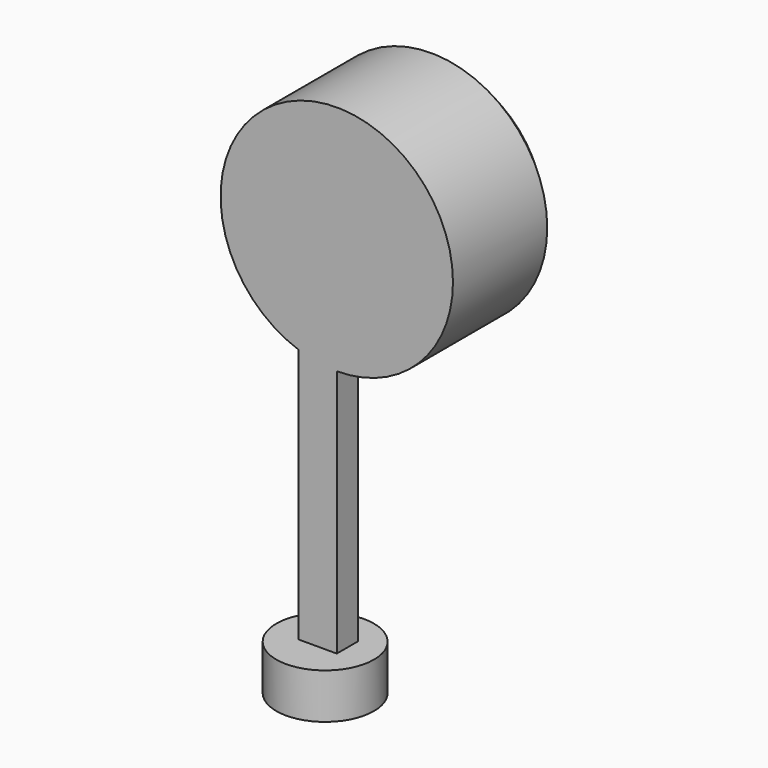
from build123d import *

# Parameters (mm, degrees)
F0_R     = 27.3478618837
F1_DEPTH = 25.4
F2_W     = 21.4937683195
F2_H     = 14.953751117
F3_DEPTH = 228.6
F4_R     = 65.1026145731
F5_DEPTH = 76.2
F6_R     = 40.595906751
F7_DEPTH = 25.4
F8_R     = 12.7


# Not quite as in the source:
# - a fillet or chamfer that OpenCascade refuses, or shapes differently, is made with other operations: its cross-section is extruded or revolved along the edge and cut away or added


with BuildPart() as f1:
    # F0 (on Top) → F1 (new body)
    with BuildSketch(Plane.XY):
        with Locations((-20.4128082842, 28.926692903)):
            Circle(F0_R)
    extrude(amount=F1_DEPTH)

    # F2 (on face) → F3 (join)
    with BuildSketch(Plane.XY.offset(25.4)):
        with Locations((-20.0721742585, 30.7035986334)):
            Rectangle(F2_W, F2_H)
    extrude(amount=F3_DEPTH)

    # F4 (on face) → F5 (join)
    with BuildSketch(Plane.XZ.offset(-23.2267230749)):
        with Locations((-9.3252900988, 229.8023849726)):
            Circle(F4_R)
    extrude(amount=-F5_DEPTH)

    # F6 (on face) → F7 (cut)
    with BuildSketch(Plane(origin=(0, 99.4267230749, 0), x_dir=(-1, 0, 0), z_dir=(0, 1, 0))):
        with Locations((30.0150513649, 226.0579317808)):
            Circle(F6_R)
    extrude(amount=-F7_DEPTH, mode=Mode.SUBTRACT)

    # F8
    f8_edges = [f1.edges().sort_by_distance(p)[0] for p in [
        (10.580855, 74.026723, 226.057932),
    ]]
    fillet(f8_edges, radius=F8_R)

    # F9: chamfer of 10.16 on 1 edges, made by hand

    # F9_s1 → F9_t2 (revolve, cut)
    with BuildSketch(Plane.XY.offset(229.8023849726)):
        Polygon((45.6173244743, 99.4267230749), (55.7773244743, 89.2667230749), (55.7773244743, 99.4267230749), align=None)
    revolve(axis=Axis((-9.3252900988, 99.4267230749, 229.8023849726), (0, -1, 0)), mode=Mode.SUBTRACT)


solid = f1.part
